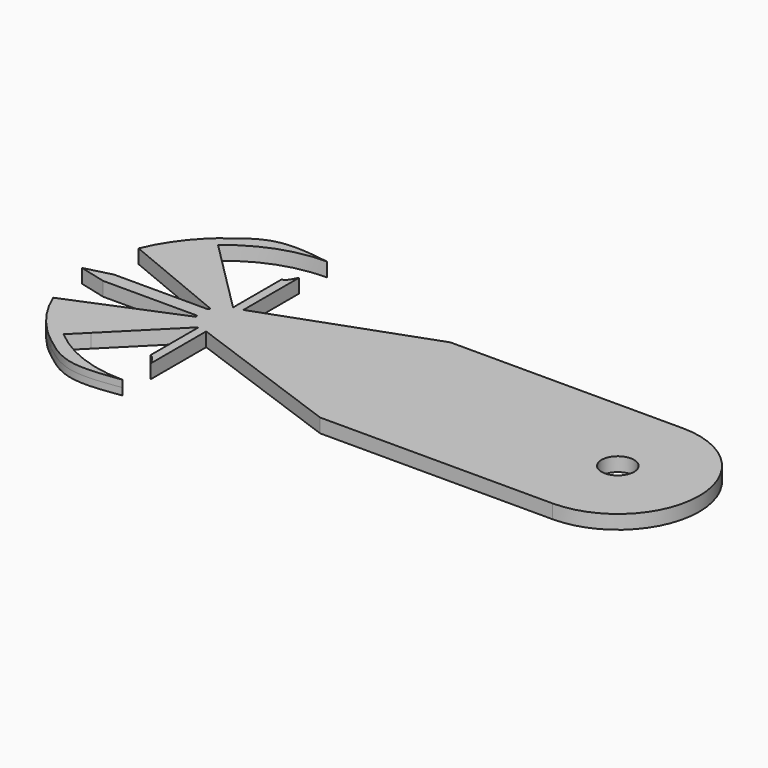
from build123d import *

# Parameters (mm, degrees)
F0_R     = 3.5
F1_DEPTH = 1.5


# Not quite as in the source:
# - a feature names something its author has since deleted; it is built from what else it names


with BuildPart() as f1:
    # F0 (on Top) → F1 (new body, symmetric)
    with BuildSketch(Plane.XY):
        with BuildLine():
            Line((-140.2163859753, 11.480502971), (-117.1193976626, 1.9134171618))
            ThreePointArc((-117.1193976626, 1.9134171618), (-117.2054191616, 1.6908667936), (-117.2807257879, 1.4644660941))
            Line((-117.2807257879, 1.4644660941), (-135.5639451435, 1.4644660941))
            Line((-135.5639451435, 1.4644660941), (-137.4212426417, 1.4644660941))
            Line((-137.4212426417, 1.4644660941), (-137.4642343313, 1.4644660941))
            Line((-137.4642343313, 1.4644660941), (-143.2, 0))
            Line((-143.2, 0), (-137.4642343313, -1.4644660941))
            Line((-137.4642343313, -1.4644660941), (-137.4212426417, -1.4644660941))
            Line((-137.4212426417, -1.4644660941), (-135.5639451435, -1.4644660941))
            Line((-135.5639451435, -1.4644660941), (-117.2807257879, -1.4644660941))
            ThreePointArc((-117.2807257879, -1.4644660941), (-117.2054191616, -1.6908667936), (-117.1193976626, -1.9134171618))
            Line((-117.1193976626, -1.9134171618), (-140.2163859753, -11.480502971))
            ThreePointArc((-140.2163859753, -11.480502971), (-137.4440883691, -16.6671069906), (-133.7132034356, -21.2132034356))
            ThreePointArc((-133.7132034356, -21.2132034356), (-133.0255631487, -21.8792426155), (-132.3170219693, -22.5230024701))
            add(Edge.make_bspline(
                [(-132.3170219693, -22.5230024701), (-131.8310141521, -22.9279318204), (-131.3450063349, -23.3328611708), (-130.8554027807, -23.7292896809)],
                knots=[0, 0, 0, 0, 0.0899480821, 0.0899480821, 0.0899480821, 0.0899480821], degree=3))
            add(Edge.make_bspline(
                [(-130.8554027807, -23.7292896809), (-128.7296529668, -25.4504941622), (-123.6181233569, -29.0879440293), (-116.5404183436, -28.0770720452), (-112.5, -27.5)],
                knots=[0.0899480821, 0.0899480821, 0.0899480821, 0.0899480821, 0.4804826627, 1, 1, 1, 1], degree=3))
            ThreePointArc((-112.5, -27.5), (-122.1329967473, -25.7576274852), (-130.5453194023, -20.7512999031))
            Line((-130.5453194023, -20.7512999031), (-127.2940194993, -17.5))
            Line((-127.2940194993, -17.5), (-114.4134171618, -4.6193976626))
            Line((-114.4134171618, -4.6193976626), (-114.4134171618, -17.6193976626))
            add(Edge.make_bspline(
                [(-114.4134171618, -17.6193976626), (-114.1696893018, -17.7059100784), (-113.5209993488, -17.936165803), (-112.89241231, -19.2067830939), (-112.5, -20)],
                knots=[0, 0, 0, 0, 0.3757231924, 1, 1, 1, 1], degree=3))
            Line((-112.5, -20), (-112.5, -5))
            Line((-112.5, -5), (-77.9963913669, -17.5))
            Line((-77.9963913669, -17.5), (-27.9963913669, -17.5))
            ThreePointArc((-27.9963913669, -17.5), (-10.4963913669, 0), (-27.9963913669, 17.5))
            Line((-27.9963913669, 17.5), (-77.9963913669, 17.5))
            Line((-77.9963913669, 17.5), (-112.5, 5))
            Line((-112.5, 5), (-112.5, 20))
            add(Edge.make_bspline(
                [(-114.4134171618, 17.6193976626), (-114.1696893018, 17.7059100784), (-113.5209993488, 17.936165803), (-112.89241231, 19.2067830939), (-112.5, 20)],
                knots=[0, 0, 0, 0, 0.3757231924, 1, 1, 1, 1], degree=3))
            Line((-114.4134171618, 17.6193976626), (-114.4134171618, 4.6193976626))
            Line((-114.4134171618, 4.6193976626), (-127.2940194993, 17.5))
            Line((-127.2940194993, 17.5), (-130.5453194023, 20.7512999031))
            ThreePointArc((-130.5453194023, 20.7512999031), (-122.1329967473, 25.7576274852), (-112.5, 27.5))
            add(Edge.make_bspline(
                [(-132.3170219693, 22.5230024701), (-129.7208762292, 24.6860450606), (-124.3176724473, 29.1878570062), (-116.5404183436, 28.0770720452), (-112.5, 27.5)],
                knots=[0, 0, 0, 0, 0.4804826627, 1, 1, 1, 1], degree=3))
            Line((-132.3170219693, 22.5230024701), (-133.7132034356, 21.2132034356))
            ThreePointArc((-133.7132034356, 21.2132034356), (-137.4440883691, 16.6671069906), (-140.2163859753, 11.480502971))
        make_face()
        with Locations((-27.9963913669, 0)):
            Circle(F0_R, mode=Mode.SUBTRACT)
    extrude(amount=F1_DEPTH, both=True)


solid = f1.part
